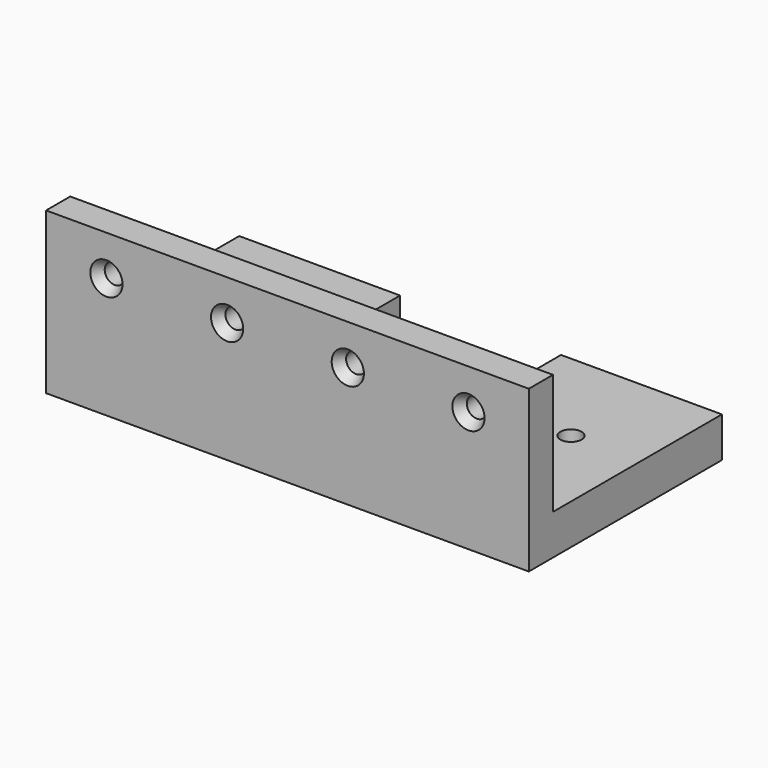
from build123d import *

# Parameters (mm, degrees)
F1_DEPTH                  = 76.2
F2_W                      = 25.4
F2_H                      = 33.3375
F3_DEPTH                  = 25.4
F4_R                      = 9.525
F5_DEPTH                  = 3.175
F6_R                      = 1.6764
F7_DEPTH                  = 25.4
F8_R                      = 1.5875
F9_DEPTH                  = 25.4
F10_R                     = 2.54
F11_DEPTH                 = 25.4
DRAFT_F11_DRAFTED_ANGLE   = 30
DRAFT_F11_2_DRAFTED_ANGLE = 30
DRAFT_F11_3_DRAFTED_ANGLE = 30
DRAFT_F11_4_DRAFTED_ANGLE = 30


# Not quite as in the source:
# - an extrude with a draft is written as a straight extrude whose walls are then drafted


with BuildPart() as f1:
    # F0 (on Right) → F1 (new body)
    with BuildSketch(Plane.YZ):
        Polygon((0, 25.4), (0, 0), (38.1, 0), (38.1, 6.35), (4.7625, 6.35), (4.7625, 25.4), align=None)
    extrude(amount=F1_DEPTH)

    # F2 (on face) → F3 (cut)
    with BuildSketch(Plane.XY.offset(6.35)):
        with Locations((38.1, 21.43125)):
            Rectangle(F2_W, F2_H)
    extrude(amount=-F3_DEPTH, mode=Mode.SUBTRACT)

    # F4 (on face) → F5 (cut)
    with BuildSketch(Plane(origin=(0, 0, 0), x_dir=(1, 0, 0), z_dir=(0, 0, -1))):
        with Locations((65.225, -22.0345)):
            Circle(F4_R)
        with Locations((10.975, -22.0345)):
            Circle(F4_R)
    extrude(amount=-F5_DEPTH, mode=Mode.SUBTRACT)

    # F6 (on face) → F7 (cut)
    with BuildSketch(Plane(origin=(0, 0, 0), x_dir=(1, 0, 0), z_dir=(0, 0, -1))):
        with Locations((65.225, -22.0345)):
            Circle(F6_R)
        with Locations((10.975, -22.0345)):
            Circle(F6_R)
    extrude(amount=-F7_DEPTH, mode=Mode.SUBTRACT)

    # F8 (on face) → F9 (cut)
    with BuildSketch(Plane.XZ):
        with Locations((9.525, 19.05)):
            Circle(F8_R)
        with Locations((28.575, 19.05)):
            Circle(F8_R)
        with Locations((47.625, 19.05)):
            Circle(F8_R)
        with Locations((66.675, 19.05)):
            Circle(F8_R)
    extrude(amount=-F9_DEPTH, mode=Mode.SUBTRACT)


with BuildPart() as f11_drafted:
    # F10 (on face) → F11 (new body)
    with BuildSketch(Plane.XZ):
        with Locations((9.525, 19.05)):
            Circle(F10_R)
    extrude(amount=-F11_DEPTH)

    # draft_F11_drafted
    draft_f11_drafted_walls = [f11_drafted.faces().sort_by_distance(p)[0] for p in [
        (6.985, 16.9333333333, 19.05),
    ]]
    draft(draft_f11_drafted_walls, neutral_plane=Plane(origin=(0, 0, 0), x_dir=(1, 0, 0), z_dir=(0, 1, 0)), angle=DRAFT_F11_DRAFTED_ANGLE)


with BuildPart() as f1_1:
    add(f1.part)

    # join_F11_drafted: cut F11_drafted
    add(f11_drafted.part, mode=Mode.SUBTRACT)


with BuildPart() as f11_2_drafted:
    # F10 (on face) → F11, piece 2 (new body)
    with BuildSketch(Plane.XZ):
        with Locations((28.575, 19.05)):
            Circle(F10_R)
    extrude(amount=-F11_DEPTH)

    # draft_F11_2_drafted
    draft_f11_2_drafted_walls = [f11_2_drafted.faces().sort_by_distance(p)[0] for p in [
        (26.035, 16.9333333333, 19.05),
    ]]
    draft(draft_f11_2_drafted_walls, neutral_plane=Plane(origin=(0, 0, 0), x_dir=(1, 0, 0), z_dir=(0, 1, 0)), angle=DRAFT_F11_2_DRAFTED_ANGLE)


with BuildPart() as f1_2:
    add(f1_1.part)

    # join_F11_2_drafted: cut F11_2_drafted
    add(f11_2_drafted.part, mode=Mode.SUBTRACT)


with BuildPart() as f11_3_drafted:
    # F10 (on face) → F11, piece 3 (new body)
    with BuildSketch(Plane.XZ):
        with Locations((47.625, 19.05)):
            Circle(F10_R)
    extrude(amount=-F11_DEPTH)

    # draft_F11_3_drafted
    draft_f11_3_drafted_walls = [f11_3_drafted.faces().sort_by_distance(p)[0] for p in [
        (45.085, 16.9333333333, 19.05),
    ]]
    draft(draft_f11_3_drafted_walls, neutral_plane=Plane(origin=(0, 0, 0), x_dir=(1, 0, 0), z_dir=(0, 1, 0)), angle=DRAFT_F11_3_DRAFTED_ANGLE)


with BuildPart() as f1_3:
    add(f1_2.part)

    # join_F11_3_drafted: cut F11_3_drafted
    add(f11_3_drafted.part, mode=Mode.SUBTRACT)


with BuildPart() as f11_4_drafted:
    # F10 (on face) → F11, piece 4 (new body)
    with BuildSketch(Plane.XZ):
        with Locations((66.675, 19.05)):
            Circle(F10_R)
    extrude(amount=-F11_DEPTH)

    # draft_F11_4_drafted
    draft_f11_4_drafted_walls = [f11_4_drafted.faces().sort_by_distance(p)[0] for p in [
        (64.135, 16.9333333333, 19.05),
    ]]
    draft(draft_f11_4_drafted_walls, neutral_plane=Plane(origin=(0, 0, 0), x_dir=(1, 0, 0), z_dir=(0, 1, 0)), angle=DRAFT_F11_4_DRAFTED_ANGLE)


with BuildPart() as f1_4:
    add(f1_3.part)

    # join_F11_4_drafted: cut F11_4_drafted
    add(f11_4_drafted.part, mode=Mode.SUBTRACT)


solid = f1_4.part
